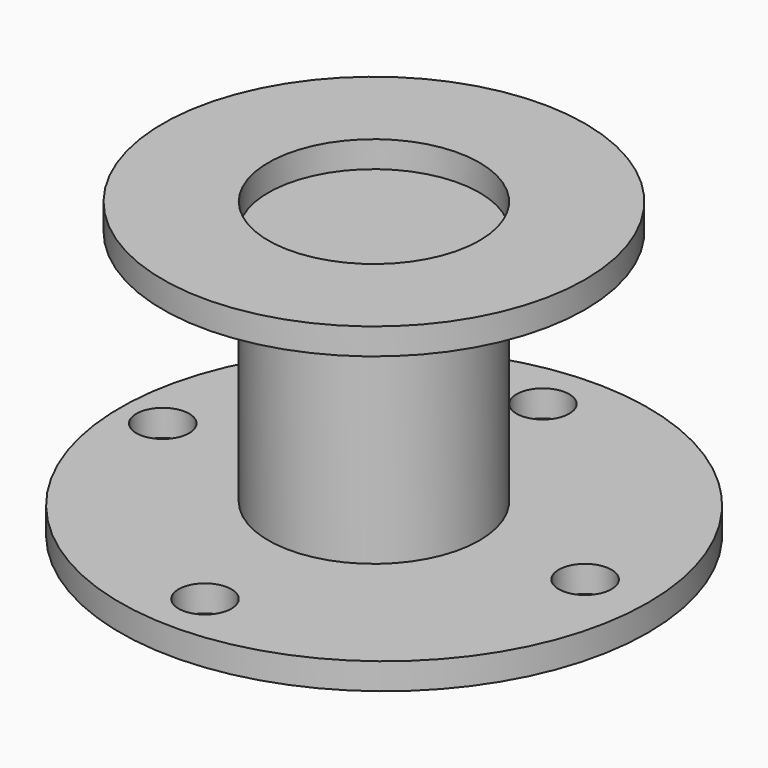
from build123d import *

# Parameters (mm, degrees)
F0_R      = 63.5
F1_DEPTH  = 6.35
F2_R      = 25.4
F3_DEPTH  = 57.15
F4_R      = 6.35
F5_DEPTH  = 25.4
F6_R      = 6.35
F7_DEPTH  = 25.4
F8_R      = 6.35
F9_DEPTH  = 25.4
F10_R     = 6.35
F11_DEPTH = 25.4
F12_R     = 50.8
F12_R_2   = 25.4
F13_DEPTH = 6.35


# Not quite as in the source:
# - a feature of the source that left no trace in its solid (it failed there, or was rolled back) is left out


with BuildPart() as f1:
    # F0 (on Top) → F1 (new body)
    with BuildSketch(Plane.XY):
        with Locations((2.4463504087, 0)):
            Circle(F0_R)
    extrude(amount=F1_DEPTH)

    # F2 (on face) → F3 (join)
    with BuildSketch(Plane.XY.offset(6.35)):
        Circle(F2_R)
    extrude(amount=F3_DEPTH)

    # F4 (on face) → F5 (cut)
    with BuildSketch(Plane.XY.offset(6.35)):
        with Locations((0, 50.8)):
            Circle(F4_R)
    extrude(amount=-F5_DEPTH, mode=Mode.SUBTRACT)

    # F6 (on face) → F7 (cut)
    with BuildSketch(Plane.XY.offset(6.35)):
        with Locations((-50.8, 0)):
            Circle(F6_R)
    extrude(amount=-F7_DEPTH, mode=Mode.SUBTRACT)

    # F8 (on face) → F9 (cut)
    with BuildSketch(Plane.XY.offset(6.35)):
        with Locations((0, -50.8)):
            Circle(F8_R)
    extrude(amount=-F9_DEPTH, mode=Mode.SUBTRACT)

    # F10 (on face) → F11 (cut)
    with BuildSketch(Plane.XY.offset(6.35)):
        with Locations((50.8, 0)):
            Circle(F10_R)
    extrude(amount=-F11_DEPTH, mode=Mode.SUBTRACT)


with BuildPart() as f13:
    # F12 (on face) → F13 (new body)
    with BuildSketch(Plane.XY.offset(63.5)):
        Circle(F12_R)
        Circle(F12_R_2, mode=Mode.SUBTRACT)
    extrude(amount=F13_DEPTH)


solid = Compound([f1.part, f13.part])
